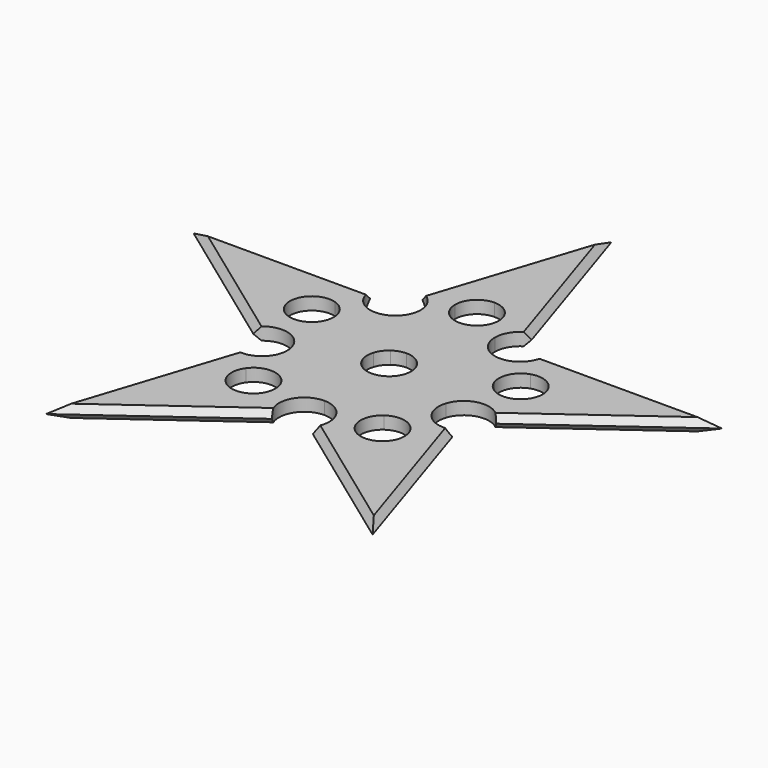
from build123d import *

# Parameters (mm, degrees)
F1_DEPTH = 6.35
F2_SIZE  = 3.17499


# Not quite as in the source:
# - a fillet or chamfer is up to 0.001 mm smaller than in the source, because OpenCascade refuses the exact size
# - a feature names something its author has since deleted; it is built from what else it names


with BuildPart() as f1:
    # F0 (on Top) → F1 (new body)
    with BuildSketch(Plane.XY):
        with BuildLine():
            Line((19.3683549781, 156.3463236885), (-8.1032558219, 71.7973993899))
            Line((-8.1032558219, 71.7973993899), (8.3683549781, 71.7973993899))
            ThreePointArc((8.3683549781, 71.7973993899), (11.590180385, 79.5755739829), (19.3683549781, 82.7973993899))
            Line((19.3683549781, 82.7973993899), (19.3683549781, 156.3463236885))
        make_face()
        with BuildLine():
            Line((19.3683549781, 60.7973993899), (19.3683549781, 59.7189816329))
            Line((19.3683549781, 59.7189816329), (38.0644816066, 59.7189816329))
            ThreePointArc((38.0644816066, 59.7189816329), (40.489965778, 67.183854337), (46.839965778, 71.7973993899))
            Line((46.839965778, 71.7973993899), (30.3683549781, 71.7973993899))
            ThreePointArc((30.3683549781, 71.7973993899), (27.1465295711, 64.0192247968), (19.3683549781, 60.7973993899))
        make_face()
        with BuildLine():
            Line((19.3683549781, 59.7189816329), (0.6722283496, 59.7189816329))
            ThreePointArc((0.6722283496, 59.7189816329), (-0.7119887932, 53.9533022862), (-4.5628989463, 49.4444658044))
            Line((-4.5628989463, 49.4444658044), (12.9027172029, 25.4051075068))
            ThreePointArc((12.9027172029, 25.4051075068), (15.96916804, 26.9675422479), (19.3683549781, 27.5059205686))
            Line((19.3683549781, 27.5059205686), (19.3683549781, 59.7189816329))
        make_face()
        with BuildLine():
            ThreePointArc((-4.5628989463, 49.4444658044), (-17.7934509971, 48.4031987757), (-24.7277716504, 59.7189816329))
            Line((-24.7277716504, 59.7189816329), (-29.8177793123, 44.0535488478))
            ThreePointArc((-29.8177793123, 44.0535488478), (-24.3177793123, 40.0575649437), (-22.2169662504, 33.5919271685))
            ThreePointArc((-22.2169662504, 33.5919271685), (-22.3523945039, 31.8711480531), (-22.7553445712, 30.1927402304))
            Line((-22.7553445712, 30.1927402304), (8.9067332988, 19.9051075068))
            ThreePointArc((8.9067332988, 19.9051075068), (10.46916804, 22.9715583438), (12.9027172029, 25.4051075068))
            Line((12.9027172029, 25.4051075068), (-4.5628989463, 49.4444658044))
        make_face()
        with BuildLine():
            Line((-36.6161531886, 23.1303054893), (-41.7061608505, 7.4648727041))
            ThreePointArc((-41.7061608505, 7.4648727041), (-29.4449273159, 12.5436419256), (-19.353227265, 3.9245158286))
            Line((-19.353227265, 3.9245158286), (8.9067332988, 13.1067336305))
            ThreePointArc((8.9067332988, 13.1067336305), (8.3683549781, 16.5059205686), (8.9067332988, 19.9051075068))
            Line((8.9067332988, 19.9051075068), (-22.7553445712, 30.1927402304))
            ThreePointArc((-22.7553445712, 30.1927402304), (-28.2230707533, 23.7908554024), (-36.6161531886, 23.1303054893))
        make_face()
        with BuildLine():
            ThreePointArc((-18.7316450219, 0), (-23.9667723178, -10.2745158286), (-35.3561608505, -12.0784177569))
            Line((-35.3561608505, -12.0784177569), (-22.0303477886, -21.7601876667))
            ThreePointArc((-22.0303477886, -21.7601876667), (-14.8519399659, -17.3612536953), (-6.6655230753, -19.3266385037))
            Line((-6.6655230753, -19.3266385037), (12.9027172029, 7.6067336305))
            ThreePointArc((12.9027172029, 7.6067336305), (10.46916804, 10.0402827934), (8.9067332988, 13.1067336305))
            Line((8.9067332988, 13.1067336305), (-19.353227265, 3.9245158286))
            ThreePointArc((-19.353227265, 3.9245158286), (-18.8880030964, 1.986717706), (-18.7316450219, 0))
        make_face()
        with BuildLine():
            ThreePointArc((19.3683549781, 5.5059205686), (15.96916804, 6.0442988894), (12.9027172029, 7.6067336305))
            Line((12.9027172029, 7.6067336305), (-6.6655230753, -19.3266385037))
            ThreePointArc((-6.6655230753, -19.3266385037), (-3.3300890844, -23.2319299447), (-2.1311608505, -28.2258254419))
            ThreePointArc((-2.1311608505, -28.2258254419), (-2.6695391712, -31.62501238), (-4.2319739124, -34.6914632171))
            Line((-4.2319739124, -34.6914632171), (9.0938391495, -44.3732331268))
            ThreePointArc((9.0938391495, -44.3732331268), (8.0525721209, -31.142681076), (19.3683549781, -24.2083604227))
            Line((19.3683549781, -24.2083604227), (19.3683549781, 5.5059205686))
        make_face()
        with BuildLine():
            Line((45.4022330314, -19.3266385037), (25.8339927533, 7.6067336305))
            ThreePointArc((25.8339927533, 7.6067336305), (22.7675419162, 6.0442988894), (19.3683549781, 5.5059205686))
            Line((19.3683549781, 5.5059205686), (19.3683549781, -24.2083604227))
            ThreePointArc((19.3683549781, -24.2083604227), (28.3486110991, -27.9281043016), (32.0683549781, -36.9083604227))
            ThreePointArc((32.0683549781, -36.9083604227), (31.446772735, -40.8328762512), (29.6428708066, -44.3732331268))
            Line((29.6428708066, -44.3732331268), (42.9686838685, -34.6914632171))
            ThreePointArc((42.9686838685, -34.6914632171), (41.0032990601, -26.5050463264), (45.4022330314, -19.3266385037))
        make_face()
        with BuildLine():
            ThreePointArc((29.8299766573, 13.1067336305), (28.2675419162, 10.0402827934), (25.8339927533, 7.6067336305))
            Line((25.8339927533, 7.6067336305), (45.4022330314, -19.3266385037))
            ThreePointArc((45.4022330314, -19.3266385037), (53.5886499221, -17.3612536953), (60.7670577448, -21.7601876667))
            Line((60.7670577448, -21.7601876667), (74.0928708066, -12.0784177569))
            ThreePointArc((74.0928708066, -12.0784177569), (61.188098857, -8.9802561211), (58.0899372211, 3.9245158286))
            Line((58.0899372211, 3.9245158286), (29.8299766573, 13.1067336305))
        make_face()
        with BuildLine():
            Line((61.4920545274, 30.1927402304), (29.8299766573, 19.9051075068))
            ThreePointArc((29.8299766573, 19.9051075068), (30.2329267246, 18.2266996841), (30.3683549781, 16.5059205686))
            ThreePointArc((30.3683549781, 16.5059205686), (30.2329267246, 14.7851414532), (29.8299766573, 13.1067336305))
            Line((29.8299766573, 13.1067336305), (58.0899372211, 3.9245158286))
            ThreePointArc((58.0899372211, 3.9245158286), (68.1816372721, 12.5436419256), (80.4428708066, 7.4648727041))
            Line((80.4428708066, 7.4648727041), (75.3528631447, 23.1303054893))
            ThreePointArc((75.3528631447, 23.1303054893), (66.9597807095, 23.7908554024), (61.4920545274, 30.1927402304))
        make_face()
        with BuildLine():
            Line((68.5544892685, 44.0535488478), (63.4644816066, 59.7189816329))
            ThreePointArc((63.4644816066, 59.7189816329), (56.5301609533, 48.4031987757), (43.2996089025, 49.4444658044))
            Line((43.2996089025, 49.4444658044), (25.8339927533, 25.4051075068))
            ThreePointArc((25.8339927533, 25.4051075068), (28.2675419162, 22.9715583438), (29.8299766573, 19.9051075068))
            Line((29.8299766573, 19.9051075068), (61.4920545274, 30.1927402304))
            ThreePointArc((61.4920545274, 30.1927402304), (62.1526044405, 38.5858226656), (68.5544892685, 44.0535488478))
        make_face()
        with BuildLine():
            Line((8.3683549781, 71.7973993899), (-8.1032558219, 71.7973993899))
            ThreePointArc((-8.1032558219, 71.7973993899), (-1.7532558219, 67.183854337), (0.6722283496, 59.7189816329))
            Line((0.6722283496, 59.7189816329), (19.3683549781, 59.7189816329))
            Line((19.3683549781, 59.7189816329), (19.3683549781, 60.7973993899))
            ThreePointArc((19.3683549781, 60.7973993899), (11.590180385, 64.0192247968), (8.3683549781, 71.7973993899))
        make_face()
        with BuildLine():
            Line((46.839965778, 71.7973993899), (19.3683549781, 156.3463236885))
            Line((19.3683549781, 156.3463236885), (19.3683549781, 82.7973993899))
            ThreePointArc((19.3683549781, 82.7973993899), (27.1465295711, 79.5755739829), (30.3683549781, 71.7973993899))
            Line((30.3683549781, 71.7973993899), (46.839965778, 71.7973993899))
        make_face()
        with BuildLine():
            Line((38.0644816066, 59.7189816329), (19.3683549781, 59.7189816329))
            Line((19.3683549781, 59.7189816329), (19.3683549781, 27.5059205686))
            ThreePointArc((19.3683549781, 27.5059205686), (22.7675419162, 26.9675422479), (25.8339927533, 25.4051075068))
            Line((25.8339927533, 25.4051075068), (43.2996089025, 49.4444658044))
            ThreePointArc((43.2996089025, 49.4444658044), (39.4486987494, 53.9533022862), (38.0644816066, 59.7189816329))
        make_face()
        with BuildLine():
            Line((-29.8177793123, 44.0535488478), (-24.7277716504, 59.7189816329))
            Line((-24.7277716504, 59.7189816329), (-113.6277716504, 59.7189816329))
            Line((-113.6277716504, 59.7189816329), (-43.6785879297, 36.9911141066))
            ThreePointArc((-43.6785879297, 36.9911141066), (-38.2108617476, 43.3929989346), (-29.8177793123, 44.0535488478))
        make_face()
        with BuildLine():
            Line((-43.6785879297, 36.9911141066), (-113.6277716504, 59.7189816329))
            Line((-113.6277716504, 59.7189816329), (-41.7061608505, 7.4648727041))
            Line((-41.7061608505, 7.4648727041), (-36.6161531886, 23.1303054893))
            ThreePointArc((-36.6161531886, 23.1303054893), (-43.0180380165, 28.5980316714), (-43.6785879297, 36.9911141066))
        make_face()
        with BuildLine():
            Line((-22.0303477886, -21.7601876667), (-35.3561608505, -12.0784177569))
            Line((-35.3561608505, -12.0784177569), (-62.8277716504, -96.6273420556))
            Line((-62.8277716504, -96.6273420556), (-19.5967986257, -37.12501238))
            ThreePointArc((-19.5967986257, -37.12501238), (-23.995732597, -29.9466045573), (-22.0303477886, -21.7601876667))
        make_face()
        with BuildLine():
            Line((-19.5967986257, -37.12501238), (-62.8277716504, -96.6273420556))
            Line((-62.8277716504, -96.6273420556), (9.0938391495, -44.3732331268))
            Line((9.0938391495, -44.3732331268), (-4.2319739124, -34.6914632171))
            ThreePointArc((-4.2319739124, -34.6914632171), (-11.410381735, -39.0903971884), (-19.5967986257, -37.12501238))
        make_face()
        with BuildLine():
            ThreePointArc((58.3335085819, -37.12501238), (50.1470916912, -39.0903971884), (42.9686838685, -34.6914632171))
            Line((42.9686838685, -34.6914632171), (29.6428708066, -44.3732331268))
            Line((29.6428708066, -44.3732331268), (101.5644816066, -96.6273420556))
            Line((101.5644816066, -96.6273420556), (58.3335085819, -37.12501238))
        make_face()
        with BuildLine():
            Line((74.0928708066, -12.0784177569), (60.7670577448, -21.7601876667))
            ThreePointArc((60.7670577448, -21.7601876667), (62.3294924859, -24.8266385037), (62.8678708066, -28.2258254419))
            ThreePointArc((62.8678708066, -28.2258254419), (61.6689425727, -33.219720939), (58.3335085819, -37.12501238))
            Line((58.3335085819, -37.12501238), (101.5644816066, -96.6273420556))
            Line((101.5644816066, -96.6273420556), (74.0928708066, -12.0784177569))
        make_face()
        with BuildLine():
            Line((80.4428708066, 7.4648727041), (152.3644816066, 59.7189816329))
            Line((152.3644816066, 59.7189816329), (82.4152978859, 36.9911141066))
            ThreePointArc((82.4152978859, 36.9911141066), (82.8182479532, 35.312706284), (82.9536762066, 33.5919271685))
            ThreePointArc((82.9536762066, 33.5919271685), (80.8528631447, 27.1262893933), (75.3528631447, 23.1303054893))
            Line((75.3528631447, 23.1303054893), (80.4428708066, 7.4648727041))
        make_face()
        with BuildLine():
            Line((152.3644816066, 59.7189816329), (63.4644816066, 59.7189816329))
            Line((63.4644816066, 59.7189816329), (68.5544892685, 44.0535488478))
            ThreePointArc((68.5544892685, 44.0535488478), (76.9475717037, 43.3929989346), (82.4152978859, 36.9911141066))
            Line((82.4152978859, 36.9911141066), (152.3644816066, 59.7189816329))
        make_face()
    extrude(amount=F1_DEPTH)

    # F2 (size 3.175 in the source; OpenCascade refuses exactly that, so slightly less here)
    f2_edges = [f1.edges().sort_by_distance(p)[0] for p in [
        (-77.666966, 33.591927, 6.35),
        (-69.177772, 59.718982, 6.35),
        (5.63255, 114.071862, 6.35),
        (33.10416, 114.071862, 6.35),
        (107.914482, 59.718982, 6.35),
        (116.403676, 33.591927, 6.35),
        (87.828676, -54.35288, 6.35),
        (65.603676, -70.500288, 6.35),
        (-26.866966, -70.500288, 6.35),
        (-49.091966, -54.35288, 6.35),
        (-26.866966, -70.500288, 0),
        (-49.091966, -54.35288, 0),
        (65.603676, -70.500288, 0),
        (87.828676, -54.35288, 0),
        (116.403676, 33.591927, 0),
        (107.914482, 59.718982, 0),
        (33.10416, 114.071862, 0),
        (5.63255, 114.071862, 0),
        (-69.177772, 59.718982, 0),
        (-77.666966, 33.591927, 0),
    ]]
    chamfer(f2_edges, length=F2_SIZE)


solid = f1.part
